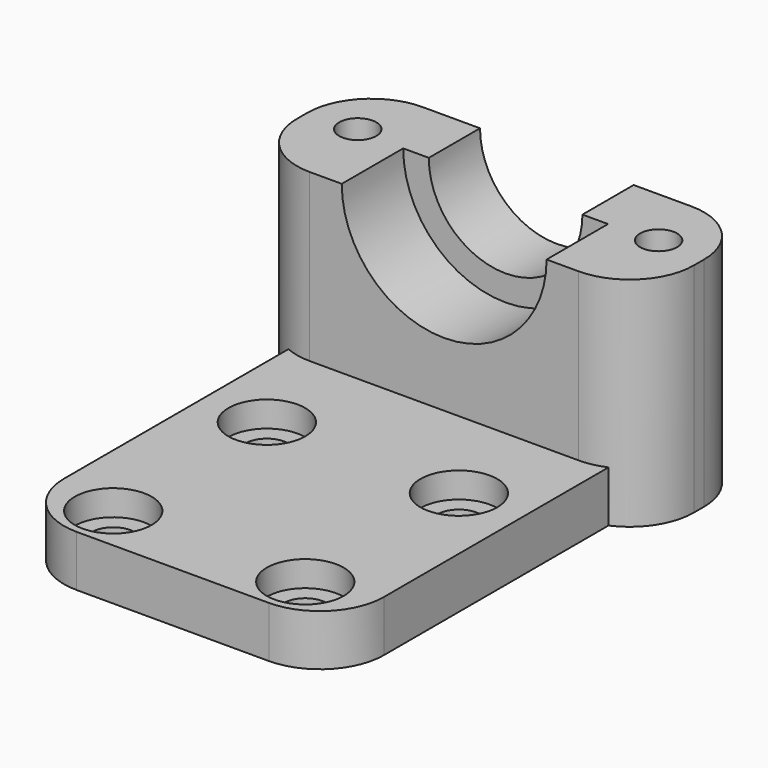
from build123d import *

# Parameters (mm, degrees)
F0_W          = 25
F0_H          = 30
F0_H_2        = 7.5
F1_DEPTH      = 4
F2_R          = 1.675
F3_DEPTH      = 25
F4_W          = 25
F4_H          = 11
F5_DEPTH      = 13
F7_DEPTH      = 6
F8_R          = 8
F9_DEPTH      = 6
F2_R_2        = 3
F10_DEPTH     = 2
F11_W         = 11
F11_H         = 17
F12_DEPTH     = 3
F13_W         = 11
F13_H         = 17
F14_DEPTH     = 3
F15_R         = 1.45
F16_DEPTH     = 25
F17_R         = 5
F18_DEPTH     = 25
F19_TEXT_SIZE = 4.1666666667
F20_DEPTH     = 1


# Not quite as in the source:
# - Text() gives the source's letters only with a copy of the font that has no kerning and outlines rounded to 1/6400 em; it was checked with that copy


with BuildPart() as f1:
    # F0 (on Top) → F1 (new body)
    with BuildSketch(Plane.XY):
        with Locations((12.5, 15)):
            Rectangle(F0_W, F0_H)
        with Locations((12.5, 33.75)):
            Rectangle(F0_W, F0_H_2)
    extrude(amount=F1_DEPTH)

    # F2 (on face) → F3 (cut)
    with BuildSketch(Plane.XY.offset(4)):
        with BuildLine():
            ThreePointArc((3.325, 18.5605346784), (5, 16.8855346784), (6.675, 18.5605346784))
            ThreePointArc((6.675, 18.5605346784), (5, 20.2355346784), (3.325, 18.5605346784))
        make_face()
        with Locations((20, 18.5605346784)):
            Circle(F2_R)
        with Locations((20, 3.5605346784)):
            Circle(F2_R)
        with Locations((5, 3.5605346784)):
            Circle(F2_R)
    extrude(amount=-F3_DEPTH, mode=Mode.SUBTRACT)

    # F4 (on face) → F5 (join)
    with BuildSketch(Plane.XY.offset(4)):
        with Locations((12.5, 32)):
            Rectangle(F4_W, F4_H)
    extrude(amount=F5_DEPTH)

    # F6 (on face) → F7 (cut)
    with BuildSketch(Plane(origin=(0, 37.5, 0), x_dir=(-1, 0, 0), z_dir=(0, 1, 0))):
        with BuildLine():
            ThreePointArc((-18.5, 17), (-12.5, 11), (-6.5, 17))
            Line((-6.5, 17), (-18.5, 17))
        make_face()
    extrude(amount=-F7_DEPTH, mode=Mode.SUBTRACT)

    # F8 (on face) → F9 (cut)
    with BuildSketch(Plane.XZ.offset(-26.5)):
        with Locations((12.5, 17)):
            Circle(F8_R)
    extrude(amount=-F9_DEPTH, mode=Mode.SUBTRACT)

    # F2 (on face) → F10 (cut)
    with BuildSketch(Plane.XY.offset(4)):
        with BuildLine():
            ThreePointArc((8, 18.5605346784), (5, 21.5605346784), (2, 18.5605346784))
            ThreePointArc((2, 18.5605346784), (5, 15.5605346784), (8, 18.5605346784))
        make_face()
        with BuildLine():
            ThreePointArc((3.325, 18.5605346784), (5, 20.2355346784), (6.675, 18.5605346784))
            ThreePointArc((6.675, 18.5605346784), (5, 16.8855346784), (3.325, 18.5605346784))
        make_face(mode=Mode.SUBTRACT)
        with Locations((20, 18.5605346784)):
            Circle(F2_R_2)
        with Locations((20, 18.5605346784)):
            Circle(F2_R, mode=Mode.SUBTRACT)
        with Locations((20, 3.5605346784)):
            Circle(F2_R_2)
        with Locations((20, 3.5605346784)):
            Circle(F2_R, mode=Mode.SUBTRACT)
        with Locations((5, 3.5605346784)):
            Circle(F2_R_2)
        with Locations((5, 3.5605346784)):
            Circle(F2_R, mode=Mode.SUBTRACT)
    extrude(amount=-F10_DEPTH, mode=Mode.SUBTRACT)

    # F11 (on face) → F12 (join)
    with BuildSketch(Plane(origin=(0, 0, 0), x_dir=(0, -1, 0), z_dir=(-1, 0, 0))):
        with Locations((-32, 8.5)):
            Rectangle(F11_W, F11_H)
    extrude(amount=F12_DEPTH)

    # F13 (on face) → F14 (join)
    with BuildSketch(Plane.YZ.offset(25)):
        with Locations((32, 8.5)):
            Rectangle(F13_W, F13_H)
    extrude(amount=F14_DEPTH)

    # F15 (on face) → F16 (cut)
    with BuildSketch(Plane.XY.offset(17)):
        with Locations((0.7499999938, 32.75)):
            Circle(F15_R)
        with Locations((24.2499999938, 32.75)):
            Circle(F15_R)
    extrude(amount=-F16_DEPTH, mode=Mode.SUBTRACT)

    # F17 (call 1 of 6: OpenCascade refuses the feature's edges together)
    f17_edges = [f1.edges().sort_by_distance(p)[0] for p in [
        (-3, 37.5, 8.5),
    ]]
    fillet(f17_edges, radius=F17_R)

    # F17#2 (call 2 of 6)
    f17_2_edges = [f1.edges().sort_by_distance(p)[0] for p in [
        (-3, 26.5, 8.5),
    ]]
    fillet(f17_2_edges, radius=F17_R)

    # F17#3 (call 3 of 6)
    f17_3_edges = [f1.edges().sort_by_distance(p)[0] for p in [
        (28, 26.5, 8.5),
    ]]
    fillet(f17_3_edges, radius=F17_R)

    # F17#4 (call 4 of 6)
    f17_4_edges = [f1.edges().sort_by_distance(p)[0] for p in [
        (28, 37.5, 8.5),
    ]]
    fillet(f17_4_edges, radius=F17_R)

    # F17#5 (call 5 of 6)
    f17_5_edges = [f1.edges().sort_by_distance(p)[0] for p in [
        (25, 0, 2),
    ]]
    fillet(f17_5_edges, radius=F17_R)

    # F17#6 (call 6 of 6)
    f17_6_edges = [f1.edges().sort_by_distance(p)[0] for p in [
        (0, 0, 2),
    ]]
    fillet(f17_6_edges, radius=F17_R)

    # F2 (on face) → F18 (cut)
    with BuildSketch(Plane.XY.offset(4)):
        with BuildLine():
            ThreePointArc((8, 18.5605346784), (5, 21.5605346784), (2, 18.5605346784))
            ThreePointArc((2, 18.5605346784), (5, 15.5605346784), (8, 18.5605346784))
        make_face()
        with BuildLine():
            ThreePointArc((3.325, 18.5605346784), (5, 20.2355346784), (6.675, 18.5605346784))
            ThreePointArc((6.675, 18.5605346784), (5, 16.8855346784), (3.325, 18.5605346784))
        make_face(mode=Mode.SUBTRACT)
        with Locations((20, 18.5605346784)):
            Circle(F2_R_2)
        with Locations((20, 18.5605346784)):
            Circle(F2_R, mode=Mode.SUBTRACT)
        with BuildLine():
            ThreePointArc((3.325, 18.5605346784), (5, 16.8855346784), (6.675, 18.5605346784))
            ThreePointArc((6.675, 18.5605346784), (5, 20.2355346784), (3.325, 18.5605346784))
        make_face()
        with Locations((20, 18.5605346784)):
            Circle(F2_R)
    extrude(amount=F18_DEPTH, mode=Mode.SUBTRACT)

    # F19 (on face) → F20 (cut)
    with BuildSketch(Plane(origin=(0, 37.5, 0), x_dir=(-1, 0, 0), z_dir=(0, 1, 0))):
        with Locations((-22.2776692708, 2)):
            Text('VOLCANO', F19_TEXT_SIZE, font='Open Sans', text_align=(TextAlign.LEFT, TextAlign.BOTTOM))
    extrude(amount=-F20_DEPTH, mode=Mode.SUBTRACT)


solid = f1.part
